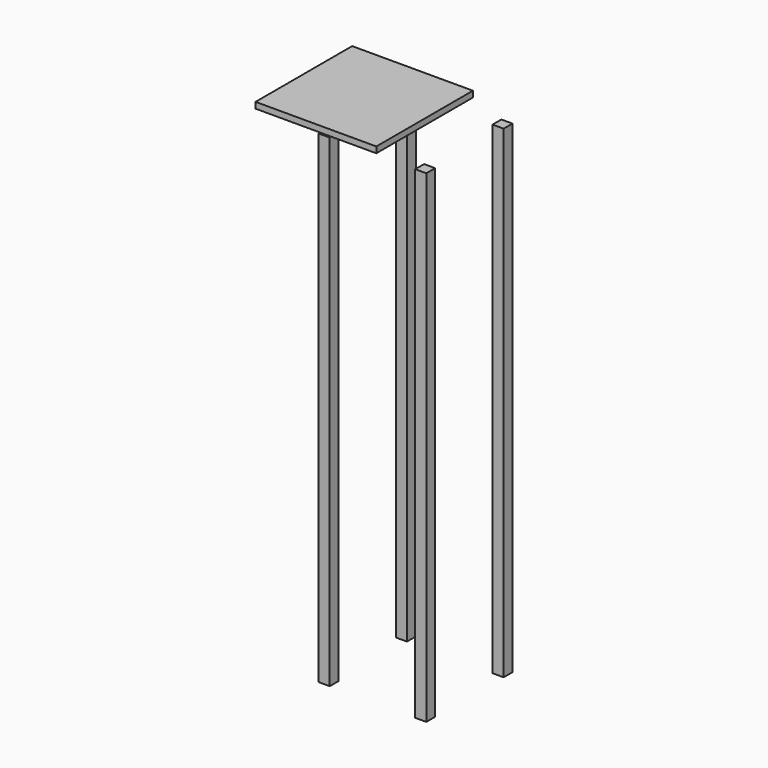
from build123d import *

# Parameters (mm, degrees)
F0_W     = 139.7
F0_H     = 139.7
F1_DEPTH = 6096
F2_W     = 1524
F2_H     = 1524
F3_DEPTH = 76.2


with BuildPart() as f1:
    # F0 (on Top) → F1 (new body)
    with BuildSketch(Plane.XY):
        with Locations((885.8353570938, -47.2469480515)):
            Rectangle(F0_W, F0_H)
    extrude(amount=F1_DEPTH)

    # F2 (on face) → F3 (join)
    with BuildSketch(Plane.XY.offset(6096)):
        with Locations((762, -549.5412114536)):
            Rectangle(F2_W, F2_H)
    extrude(amount=F3_DEPTH)


with BuildPart() as f1b:
    # F0 (on Top) → F1, piece 2 (new body)
    with BuildSketch(Plane.XY):
        with Locations((2105.0353570938, -47.2469480515)):
            Rectangle(F0_W, F0_H)
    extrude(amount=F1_DEPTH)


with BuildPart() as f1c:
    # F0 (on Top) → F1, piece 3 (new body)
    with BuildSketch(Plane.XY):
        with Locations((2105.0353570938, -1266.4469480515)):
            Rectangle(F0_W, F0_H)
    extrude(amount=F1_DEPTH)


with BuildPart() as f1d:
    # F0 (on Top) → F1, piece 4 (new body)
    with BuildSketch(Plane.XY):
        with Locations((885.8353570938, -1266.4469480515)):
            Rectangle(F0_W, F0_H)
    extrude(amount=F1_DEPTH)


solid = Compound([f1.part, f1b.part, f1c.part, f1d.part])
